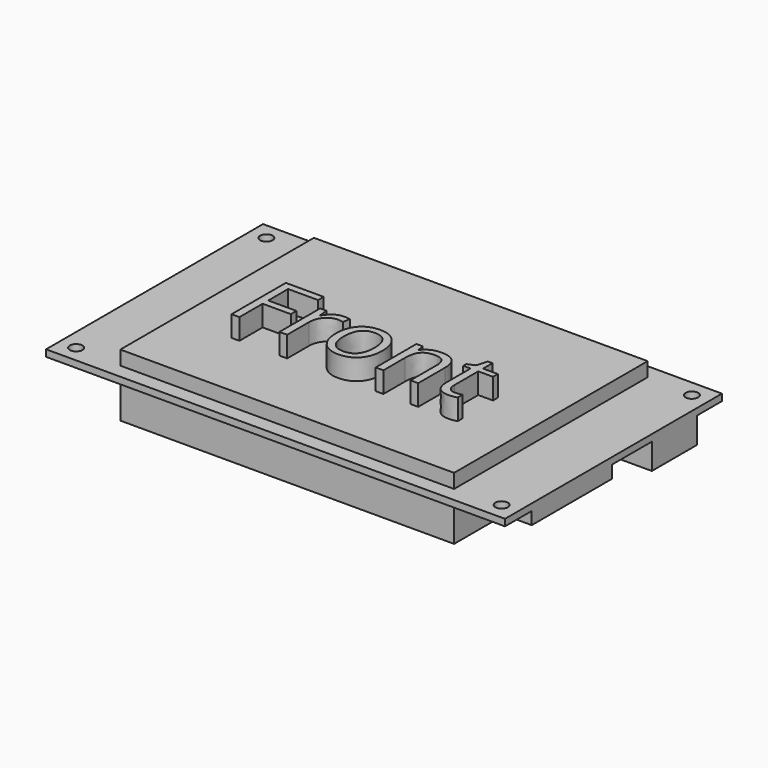
from build123d import *

# Parameters (mm, degrees)
F0_W         = 110
F0_H         = 65
F0_R         = 1.5
F0_W_2       = 80
F0_H_2       = 58
F1_DEPTH     = 1.6
F2_DEPTH     = 5
F3_DEPTH     = 10
F4_TEXT_SIZE = 22.7908164056
F5_DEPTH     = 5
F6_W         = 15
F6_H         = 13.5
F7_DEPTH     = 6.2
F6_H_2       = 24
F8_DEPTH     = 3


# Not quite as in the source:
# - Text() gives the source's letters only with a copy of the font that has no kerning and outlines rounded to 1/6400 em; it was checked with that copy


with BuildPart() as f1:
    # F0 (on Top) → F1 (new body)
    with BuildSketch(Plane.XY):
        with Locations((0, -4.0998587116)):
            Rectangle(F0_W, F0_H)
        with Locations((-51, -32.5998587116)):
            Circle(F0_R, mode=Mode.SUBTRACT)
        with Locations((51, -32.5998587116)):
            Circle(F0_R, mode=Mode.SUBTRACT)
        with Locations((0, -4.0998587116)):
            Rectangle(F0_W_2, F0_H_2, mode=Mode.SUBTRACT)
        with Locations((-51, 24.4001412884)):
            Circle(F0_R, mode=Mode.SUBTRACT)
        with Locations((51, 24.4001412884)):
            Circle(F0_R, mode=Mode.SUBTRACT)
    extrude(amount=F1_DEPTH)

    # F0 (on Top) → F2 (join)
    with BuildSketch(Plane.XY):
        with Locations((0, -4.0998587116)):
            Rectangle(F0_W_2, F0_H_2)
    extrude(amount=F2_DEPTH)

    # F0 (on Top) → F3 (join)
    with BuildSketch(Plane.XY):
        with Locations((0, -4.0998587116)):
            Rectangle(F0_W_2, F0_H_2)
    extrude(amount=-F3_DEPTH)

    # F4 (on face) → F5 (join)
    with BuildSketch(Plane.XY.offset(5)):
        with Locations((-28.9336536399, -16.409387812)):
            Text('Front', F4_TEXT_SIZE, font='Open Sans', text_align=(TextAlign.LEFT, TextAlign.BOTTOM))
    extrude(amount=F5_DEPTH)

    # F6 (on face) → F7 (join)
    with BuildSketch(Plane.XY):
        with Locations((47.5, 14.1501412884)):
            Rectangle(F6_W, F6_H)
    extrude(amount=-F7_DEPTH)

    # F6 (on face) → F8 (join)
    with BuildSketch(Plane.XY):
        with Locations((47.5, -16.5998587116)):
            Rectangle(F6_W, F6_H_2)
    extrude(amount=-F8_DEPTH)


solid = f1.part
